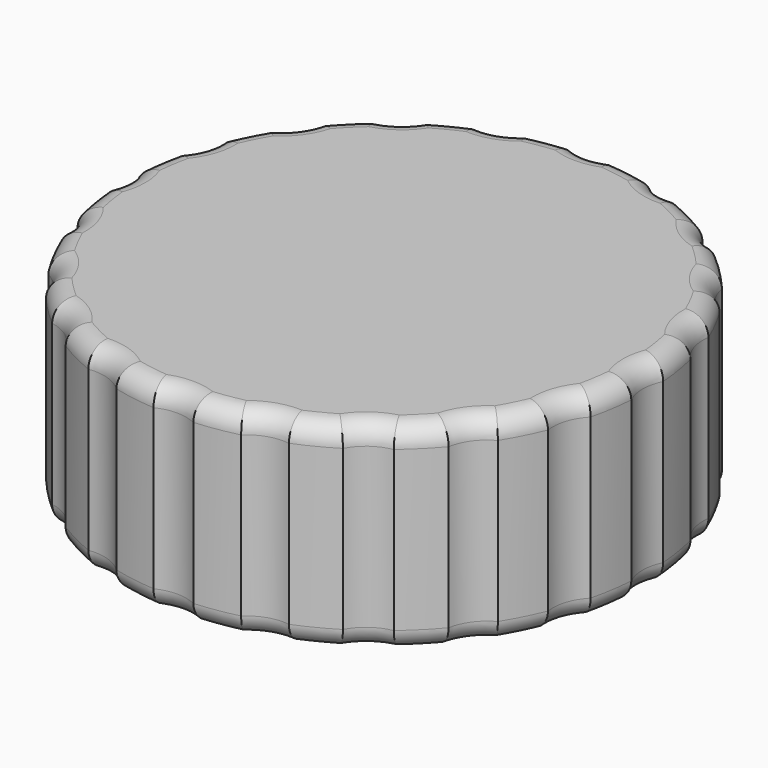
from build123d import *

# Parameters (mm, degrees)
F0_R            = 13.25
F1_DEPTH        = 10
F3_DEPTH        = 10.001
F3_COPIES_COUNT = 20
F5_R            = 1
F6_R            = 10.25
F7_DEPTH        = 5


# Not quite as in the source:
# - a pattern or mirror of a feature is missing from the dataset's text; its kind, count and spacing are read off the source's solid


with BuildPart() as f1:
    # F0 (on Top) → F1 (new body)
    with BuildSketch(Plane.XY):
        Circle(F0_R)
    extrude(amount=-F1_DEPTH)

    # F2 (on face) → F3 (cut, through all)
    with BuildSketch(Plane.XY):
        with BuildLine():
            ThreePointArc((1, 13.2122102617), (0, 13.25), (-1, 13.2122102617))
            ThreePointArc((-1, 13.2122102617), (0, 12.9800689399), (1, 13.2122102617))
        make_face()
        with BuildLine():
            ThreePointArc((1, 13.2122102617), (1.9264628309, 14.0494468031), (2.2699310601, 15.25))
            ThreePointArc((2.2699310601, 15.25), (-1.2005531969, 17.1764628309), (-1, 13.2122102617))
            ThreePointArc((-1, 13.2122102617), (0, 13.25), (1, 13.2122102617))
        make_face()
    f3 = extrude(amount=-F3_DEPTH, mode=Mode.SUBTRACT)

    # F3_copies: F3 ×20 about axis
    f3_copies_axis = Axis((0, 0, 0), (0, 0, 1))
    for i in range(1, F3_COPIES_COUNT):
        add(f3.rotate(f3_copies_axis, i * 360 / F3_COPIES_COUNT), mode=Mode.SUBTRACT)

    # F5
    f5_edges = [f1.edges().sort_by_distance(p)[0] for p in [
        (0, 12.980069, 0),
        (2.072757, 13.086871, 0),
        (4.011062, 12.344779, 0),
        (6.015374, 11.805836, 0),
        (7.629493, 10.501096, 0),
        (9.369165, 9.369165, 0),
        (10.501096, 7.629493, 0),
        (11.805836, 6.015374, 0),
        (12.344779, 4.011062, 0),
        (13.086871, 2.072757, 0),
        (12.980069, 0, 0),
        (13.086871, -2.072757, 0),
        (12.344779, -4.011062, 0),
        (11.805836, -6.015374, 0),
        (10.501096, -7.629493, 0),
        (9.369165, -9.369165, 0),
        (7.629493, -10.501096, 0),
        (6.015374, -11.805836, 0),
        (4.011062, -12.344779, 0),
        (2.072757, -13.086871, 0),
        (0, -12.980069, 0),
        (-2.072757, -13.086871, 0),
        (-4.011062, -12.344779, 0),
        (-6.015374, -11.805836, 0),
        (-7.629493, -10.501096, 0),
        (-9.369165, -9.369165, 0),
        (-10.501096, -7.629493, 0),
        (-11.805836, -6.015374, 0),
        (-12.344779, -4.011062, 0),
        (-13.086871, -2.072757, 0),
        (-12.980069, 0, 0),
        (-13.086871, 2.072757, 0),
        (-12.344779, 4.011062, 0),
        (-11.805836, 6.015374, 0),
        (-10.501096, 7.629493, 0),
        (-9.369165, 9.369165, 0),
        (-7.629493, 10.501096, 0),
        (-6.015374, 11.805836, 0),
        (-4.011062, 12.344779, 0),
        (-2.072757, 13.086871, 0),
        (0, 12.980069, -10),
        (2.072757, 13.086871, -10),
        (4.011062, 12.344779, -10),
        (6.015374, 11.805836, -10),
        (7.629493, 10.501096, -10),
        (9.369165, 9.369165, -10),
        (10.501096, 7.629493, -10),
        (11.805836, 6.015374, -10),
        (12.344779, 4.011062, -10),
        (13.086871, 2.072757, -10),
        (12.980069, 0, -10),
        (13.086871, -2.072757, -10),
        (12.344779, -4.011062, -10),
        (11.805836, -6.015374, -10),
        (10.501096, -7.629493, -10),
        (9.369165, -9.369165, -10),
        (7.629493, -10.501096, -10),
        (6.015374, -11.805836, -10),
        (4.011062, -12.344779, -10),
        (2.072757, -13.086871, -10),
        (0, -12.980069, -10),
        (-2.072757, -13.086871, -10),
        (-4.011062, -12.344779, -10),
        (-6.015374, -11.805836, -10),
        (-7.629493, -10.501096, -10),
        (-9.369165, -9.369165, -10),
        (-10.501096, -7.629493, -10),
        (-11.805836, -6.015374, -10),
        (-12.344779, -4.011062, -10),
        (-13.086871, -2.072757, -10),
        (-12.980069, 0, -10),
        (-13.086871, 2.072757, -10),
        (-12.344779, 4.011062, -10),
        (-11.805836, 6.015374, -10),
        (-10.501096, 7.629493, -10),
        (-9.369165, 9.369165, -10),
        (-7.629493, 10.501096, -10),
        (-6.015374, 11.805836, -10),
        (-4.011062, 12.344779, -10),
        (-2.072757, 13.086871, -10),
    ]]
    fillet(f5_edges, radius=F5_R)

    # F6 (on face) → F7 (cut)
    with BuildSketch(Plane(origin=(0, 0, -10), x_dir=(1, 0, 0), z_dir=(0, 0, -1))):
        Circle(F6_R)
    extrude(amount=-F7_DEPTH, mode=Mode.SUBTRACT)


solid = f1.part
